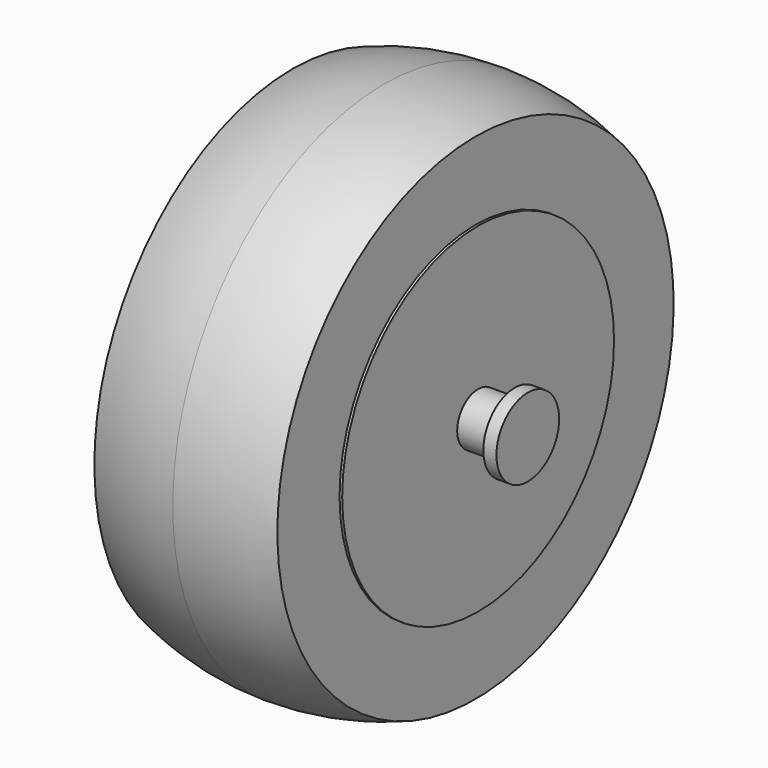
from build123d import *

# Parameters (mm, degrees)
F1_DEPTH = 17.5
F2_DEPTH = 18
F5_DEPTH = 25
F6_R     = 7.5
F7_DEPTH = 2.5
F8_R     = 7.5
F9_DEPTH = 2.5


# Not quite as in the source:
# - a feature names something its author has since deleted; it is built from what else it names


with BuildPart() as f1:
    # F0 (on Right) → F1 (new body, symmetric)
    with BuildSketch(Plane.YZ):
        with BuildLine():
            ThreePointArc((0, 50.5), (-35.7088924499, -35.7088924499), (50.5, 0))
            ThreePointArc((50.5, 0), (35.7088924499, 35.7088924499), (0, 50.5))
        make_face()
        with BuildLine():
            ThreePointArc((35, 0), (-24.7487373415, -24.7487373415), (0, 35))
            ThreePointArc((0, 35), (24.7487373415, 24.7487373415), (35, 0))
        make_face(mode=Mode.SUBTRACT)
        with BuildLine():
            ThreePointArc((35, 0), (24.7487373415, 24.7487373415), (0, 35))
            ThreePointArc((0, 35), (-24.7487373415, -24.7487373415), (35, 0))
        make_face()
        with BuildLine():
            ThreePointArc((32.5, 0), (-22.9809703886, -22.9809703886), (0, 32.5))
            ThreePointArc((0, 32.5), (22.9809703886, 22.9809703886), (32.5, 0))
        make_face(mode=Mode.SUBTRACT)
        with BuildLine():
            ThreePointArc((32.5, 0), (22.9809703886, 22.9809703886), (0, 32.5))
            ThreePointArc((0, 32.5), (-22.9809703886, -22.9809703886), (32.5, 0))
        make_face()
        with BuildLine():
            ThreePointArc((5, 0), (-3.5355339059, -3.5355339059), (0, 5))
            ThreePointArc((0, 5), (3.5355339059, 3.5355339059), (5, 0))
        make_face(mode=Mode.SUBTRACT)
    extrude(amount=F1_DEPTH, both=True)

    # F0 (on Right) → F2 (join, symmetric)
    with BuildSketch(Plane.YZ):
        with BuildLine():
            ThreePointArc((32.5, 0), (22.9809703886, 22.9809703886), (0, 32.5))
            ThreePointArc((0, 32.5), (-22.9809703886, -22.9809703886), (32.5, 0))
        make_face()
        with BuildLine():
            ThreePointArc((5, 0), (-3.5355339059, -3.5355339059), (0, 5))
            ThreePointArc((0, 5), (3.5355339059, 3.5355339059), (5, 0))
        make_face(mode=Mode.SUBTRACT)
    extrude(amount=F2_DEPTH, both=True)

    # F3 (on Front) → F4 (revolve, cut)
    with BuildSketch(Plane.XZ):
        with BuildLine():
            ThreePointArc((-17.5, 47.3708771293), (-8.888776771, 49.7115645249), (0, 50.5))
            Line((0, 50.5), (-17.5, 50.5))
            Line((-17.5, 50.5), (-17.5, 47.3708771293))
        make_face()
        with BuildLine():
            Line((17.5, 50.5), (0, 50.5))
            ThreePointArc((0, 50.5), (8.888776771, 49.7115645249), (17.5, 47.3708771293))
            Line((17.5, 47.3708771293), (17.5, 50.5))
        make_face()
    revolve(axis=Axis((-0.1237622588, 0, 0), (1, 0, 0)), mode=Mode.SUBTRACT)


with BuildPart() as f5:
    # F0 (on Right) → F5 (new body, symmetric)
    with BuildSketch(Plane.YZ):
        with BuildLine():
            ThreePointArc((5, 0), (3.5355339059, 3.5355339059), (0, 5))
            ThreePointArc((0, 5), (-3.5355339059, -3.5355339059), (5, 0))
        make_face()
    extrude(amount=F5_DEPTH, both=True)

    # F6 (on face) → F7 (join)
    with BuildSketch(Plane.YZ.offset(25)):
        Circle(F6_R)
        with BuildLine():
            ThreePointArc((5, 0), (-3.5355339059, -3.5355339059), (0, 5))
            ThreePointArc((0, 5), (3.5355339059, 3.5355339059), (5, 0))
        make_face(mode=Mode.SUBTRACT)
        with BuildLine():
            ThreePointArc((5, 0), (3.5355339059, 3.5355339059), (0, 5))
            ThreePointArc((0, 5), (-3.5355339059, -3.5355339059), (5, 0))
        make_face()
    extrude(amount=F7_DEPTH)

    # F8 (on face) → F9 (join)
    with BuildSketch(Plane(origin=(-25, 0, 0), x_dir=(0, -1, 0), z_dir=(-1, 0, 0))):
        Circle(F8_R)
        with BuildLine():
            ThreePointArc((0, 5), (3.5355339059, -3.5355339059), (-5, 0))
            ThreePointArc((-5, 0), (-3.5355339059, 3.5355339059), (0, 5))
        make_face(mode=Mode.SUBTRACT)
        with BuildLine():
            ThreePointArc((0, 5), (-3.5355339059, 3.5355339059), (-5, 0))
            ThreePointArc((-5, 0), (3.5355339059, -3.5355339059), (0, 5))
        make_face()
    extrude(amount=F9_DEPTH)


solid = Compound([f1.part, f5.part])
